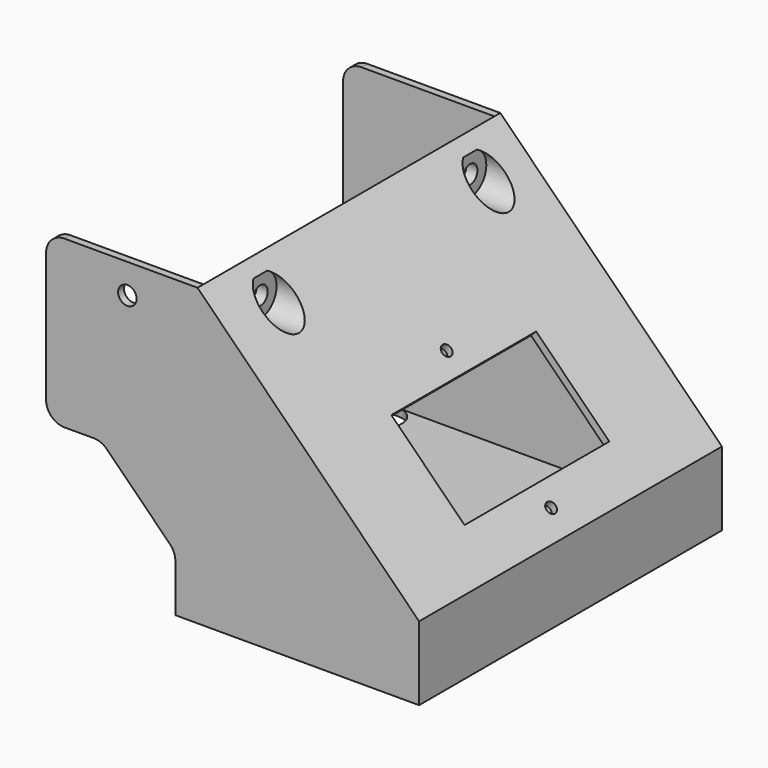
from build123d import *

# Parameters (mm, degrees)
F1_DEPTH  = 102.5
F2_T      = -2
F3_W      = 41
F3_H      = 98.5
F4_DEPTH  = 78.001
F5_W      = 98.5
F5_H      = 21.1715728753
F8_D      = 5
F9_W      = 28
F9_H      = 49
F10_DEPTH = 44.4274068712
F12_D     = 5
F12_DEPTH = 2.001
F14_D     = 3
F14_DEPTH = 12
F14_TIP   = 0.9012909285
F15_W     = 98.5
F15_H     = 2
F16_DEPTH = 20
F18_DEPTH = 25
F20_R     = 5.5
F21_DEPTH = 25
F22_R     = 5


with BuildPart() as f1:
    # F0 (on Front) → F1 (new body)
    with BuildSketch(Plane.XZ):
        Polygon((0, 80), (0, 0), (101, 0), (101, 20), (41, 80), align=None)
    extrude(amount=F1_DEPTH)

    # F2
    f2_openings = [f1.faces().sort_by_distance(p)[0] for p in [
        (0, -51.25, 40),
        (20.5, -51.25, 80),
    ]]
    offset(amount=F2_T, openings=f2_openings)

    # F3 (on face) → F4 (cut, through all)
    with BuildSketch(Plane.XY.offset(2)):
        with Locations((20.5, -51.25)):
            Rectangle(F3_W, F3_H)
    extrude(amount=F4_DEPTH, mode=Mode.SUBTRACT)

    # F5 (on face) → F6 (join, up to the last surface of F1)
    with BuildSketch(Plane(origin=(41, 0, 0), x_dir=(0, -1, 0), z_dir=(-1, 0, 0))):
        with Locations((51.25, 66.5857864376)):
            Rectangle(F5_W, F5_H)
    extrude(until=Until.LAST, dir=(1, 0, 0))

    # F8 (through all)
    with Locations(Plane(origin=(41, 0, 0), x_dir=(0, -1, 0), z_dir=(-1, 0, 0))):
        with Locations((85, 72), (14, 72)):
            Hole(F8_D / 2)

    # F9 (on face) → F10 (cut, through all)
    with BuildSketch(Plane(origin=(59.0857864376, 0, 59.0857864376), x_dir=(0.7071067812, 0, -0.7071067812), z_dir=(-0.7071067812, 0, -0.7071067812))):
        with Locations((30.405591591, 51.25)):
            Rectangle(F9_W, F9_H)
    extrude(amount=-F10_DEPTH, mode=Mode.SUBTRACT)

    # F12 (through all, one way)
    with BuildSketch(Plane(origin=(0, -100.5, 0), x_dir=(-1, 0, 0), z_dir=(0, 1, 0))):
        with Locations((-22, 72)):
            Circle(F12_D / 2)
    extrude(amount=-F12_DEPTH, mode=Mode.SUBTRACT)

    # F14
    with Locations(Plane(origin=(60.5, 0, 60.5), x_dir=(0.7071067812, 0, -0.7071067812), z_dir=(0.7071067812, 0, 0.7071067812))):
        with Locations((10.405591591, -51.75), (50.405591591, -51.75)):
            Hole(F14_D / 2, depth=F14_DEPTH)
            with Locations((0, 0, -(F14_DEPTH + F14_TIP / 2))):  # 118° drill point
                Cone(0, F14_D / 2, F14_TIP, mode=Mode.SUBTRACT)

    # F15 (on face) → F16 (cut)
    with BuildSketch(Plane(origin=(0, 0, 0), x_dir=(0, -1, 0), z_dir=(-1, 0, 0))):
        with Locations((51.25, 1)):
            Rectangle(F15_W, F15_H)
    extrude(amount=-F16_DEPTH, mode=Mode.SUBTRACT)

    # F17 (on face) → F18 (cut)
    with BuildSketch(Plane.XZ.offset(102.5)):
        Polygon((0, 35), (0, 0), (35, 0), (35, 15), (15, 35), align=None)
    extrude(amount=-F18_DEPTH, mode=Mode.SUBTRACT)

    # F20 (on offset) → F21 (cut)
    with BuildSketch(Plane(origin=(44, 0, 0), x_dir=(0, -1, 0), z_dir=(-1, 0, 0))):
        with Locations((85, 72)):
            Circle(F20_R)
        with Locations((14, 72)):
            Circle(F20_R)
    extrude(amount=-F21_DEPTH, mode=Mode.SUBTRACT)

    # F22
    f22_edges = [f1.edges().sort_by_distance(p)[0] for p in [
        (35, -77.5, 1),
        (35, -101.5, 15),
        (15, -101.5, 35),
        (20, -77.5, 1),
        (20, -2, 1),
        (0, -1, 80),
        (0, -101.5, 80),
        (0, -101.5, 35),
    ]]
    fillet(f22_edges, radius=F22_R)


solid = f1.part
